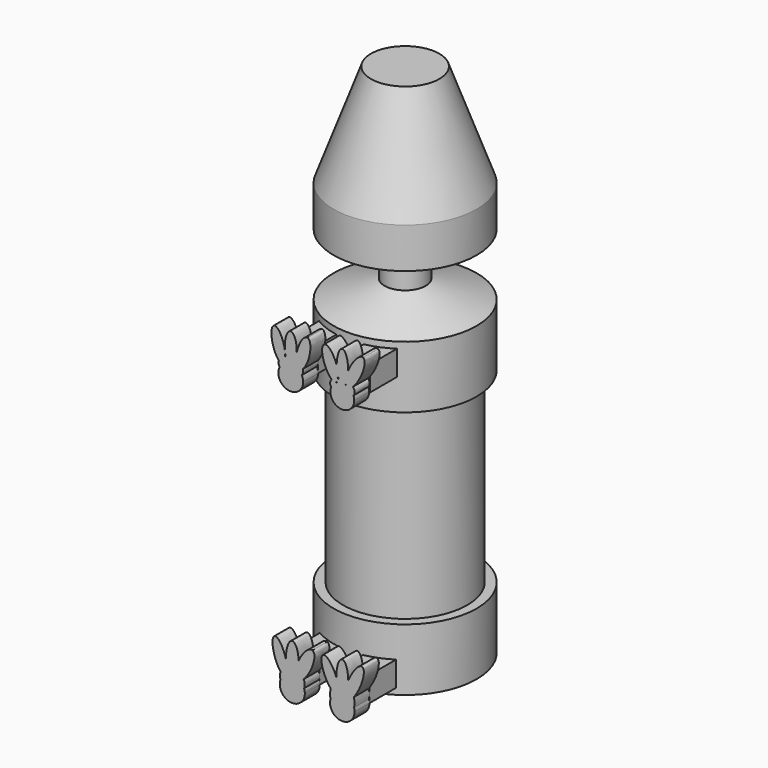
from build123d import *

# Parameters (mm, degrees)
F0_R         = 10
F1_DEPTH     = 40
F2_R         = 11.5
F2_R_2       = 10
F3_DEPTH     = 5
F4_DEPTH     = 5
F5_R         = 11.5
F6_DEPTH     = 5
F7_DEPTH     = 5
F8_W         = 4
F8_H         = 15
F9_DEPTH     = 4
F11_DEPTH    = 3
F12_R        = 11.5
F13_DEPTH    = 3
F13_TAPER    = 70
F14_R        = 3.3
F15_DEPTH    = 5
F16_R        = 11.5
F17_DEPTH    = 25
F18_S5_R     = 3.3
F18_T6_DEPTH = 18
F19_SIZE2    = 16.4848645167
F19_SIZE     = 6
F20_W        = 4
F20_H        = 15
F21_DEPTH    = 4
F23_DEPTH    = 3


# Not quite as in the source:
# - a fillet or chamfer that OpenCascade refuses, or shapes differently, is made with other operations: its cross-section is extruded or revolved along the edge and cut away or added


with BuildPart() as f1:
    # F0 (on Top) → F1 (new body)
    with BuildSketch(Plane.XY):
        Circle(F0_R)
    extrude(amount=F1_DEPTH)

    # F2 (on face) → F3 (join)
    with BuildSketch(Plane.XY.offset(40)):
        Circle(F2_R)
        Circle(F2_R_2, mode=Mode.SUBTRACT)
        Circle(F2_R_2)
    extrude(amount=F3_DEPTH)

    # F4 (add): a face of the model
    f4_faces = [f1.faces().sort_by_distance(p)[0] for p in [
        (-11.1747308807, 0, 40),
    ]]
    extrude(f4_faces, amount=F4_DEPTH)

    # F5 (on face) → F6 (join)
    with BuildSketch(Plane(origin=(0, 0, 0), x_dir=(1, 0, 0), z_dir=(0, 0, -1))):
        Circle(F5_R)
    extrude(amount=F6_DEPTH)

    # F7 (add): a face of the model
    f7_faces = [f1.faces().sort_by_distance(p)[0] for p in [
        (-11.1747308807, 0, 0),
    ]]
    extrude(f7_faces, amount=F7_DEPTH)

    # F8 (on face) → F9 (join)
    with BuildSketch(Plane.XY.offset(40)):
        with Locations((-3.98677176, -7.5)):
            Rectangle(F8_W, F8_H)
        with Locations((4.356082975, -7.5)):
            Rectangle(F8_W, F8_H)
    extrude(amount=F9_DEPTH)

    # F10 (on face) → F11 (join)
    with BuildSketch(Plane.XZ.offset(15)):
        with BuildLine():
            Line((-5.9773173295, 40), (-1.9962261905, 40))
            ThreePointArc((-1.9962261905, 40), (-2.0492726634, 40.4564744405), (-2.2055847885, 40.8886195119))
            add(Edge.make_bspline(
                [(-5.7679587315, 40.8886195119), (-3.98677176, 38.3892921565), (-2.2055847885, 40.8886195119)],
                knots=[0.4528610744, 0.4528610744, 0.4528610744, 2.6887315792, 2.6887315792, 2.6887315792], degree=2, weights=[1, 0.4375399965, 1]))
            ThreePointArc((-5.7679587315, 40.8886195119), (-5.9242708566, 40.4564744405), (-5.9773173295, 40))
        make_face()
        with BuildLine():
            ThreePointArc((-5.9773173295, 40), (-3.98677176, 38.0094544305), (-1.9962261905, 40))
            Line((-1.9962261905, 40), (-5.9773173295, 40))
        make_face()
        with BuildLine():
            add(Edge.make_bspline(
                [(-5.7679587315, 40.8886195119), (-3.98677176, 38.3892921565), (-2.2055847885, 40.8886195119)],
                knots=[0.4528610744, 0.4528610744, 0.4528610744, 2.6887315792, 2.6887315792, 2.6887315792], degree=2, weights=[1, 0.4375399965, 1]))
            ThreePointArc((-2.2055847885, 40.8886195119), (-2.4454357289, 41.2595852109), (-2.7611983029, 41.5685156567))
            add(Edge.make_bspline(
                [(-2.8505101546, 41.6343748739), (-2.8082853314, 41.5943261618), (-2.7611983029, 41.5685156567)],
                knots=[2.9464988752, 2.9464988752, 2.9464988752, 3.055351451, 3.055351451, 3.055351451], degree=2, weights=[1, 0.9985192552, 1]))
            ThreePointArc((-2.8505101546, 41.6343748739), (-3.1356310181, 41.7993974274), (-3.4440645683, 41.9151346084))
            add(Edge.make_bspline(
                [(-4.5294789517, 41.9151346084), (-3.98677176, 40.9549701782), (-3.4440645683, 41.9151346084)],
                knots=[2.5453526146, 2.5453526146, 2.5453526146, 3.7378326925, 3.7378326925, 3.7378326925], degree=2, weights=[1, 0.8274528096, 1]))
            ThreePointArc((-4.5294789517, 41.9151346084), (-5.2570293446, 41.5325525547), (-5.7679587315, 40.8886195119))
        make_face()
        with BuildLine():
            ThreePointArc((-2.7611983029, 41.5685156567), (-2.4454357289, 41.2595852109), (-2.2055847885, 40.8886195119))
            add(Edge.make_bspline(
                [(-2.2055847885, 40.8886195119), (-1.894765034, 41.324755823), (-2.0607312879, 41.7963605451)],
                knots=[2.6887315792, 2.6887315792, 2.6887315792, 3.3774021712, 3.3774021712, 3.3774021712], degree=2, weights=[1, 0.9413000454, 1]))
            add(Edge.make_bspline(
                [(-2.7611983029, 41.5685156567), (-2.4618498874, 41.4044294098), (-2.0607312879, 41.7963605451)],
                knots=[3.055351451, 3.055351451, 3.055351451, 3.7221879744, 3.7221879744, 3.7221879744], degree=2, weights=[1, 0.9449291548, 1]))
        make_face()
        with BuildLine():
            ThreePointArc((-2.8505101546, 41.6343748739), (-2.8053952008, 41.6020677544), (-2.7611983029, 41.5685156567))
            add(Edge.make_bspline(
                [(-2.7611983029, 41.5685156567), (-2.4618498874, 41.4044294098), (-2.0607312879, 41.7963605451)],
                knots=[3.055351451, 3.055351451, 3.055351451, 3.7221879744, 3.7221879744, 3.7221879744], degree=2, weights=[1, 0.9449291548, 1]))
            add(Edge.make_bspline(
                [(-2.0607312879, 41.7963605451), (-2.283512479, 42.4294088862), (-3.1471861713, 42.7053627261)],
                knots=[3.3774021712, 3.3774021712, 3.3774021712, 4.2746981663, 4.2746981663, 4.2746981663], degree=2, weights=[1, 0.9010343537, 1]))
            add(Edge.make_bspline(
                [(-3.1471861713, 42.7053627261), (-3.142060161, 41.910899472), (-2.8505101546, 41.6343748739)],
                knots=[2.2269084938, 2.2269084938, 2.2269084938, 2.9464988752, 2.9464988752, 2.9464988752], degree=2, weights=[1, 0.9359689531, 1]))
        make_face()
        with BuildLine():
            add(Edge.make_bspline(
                [(-5.9676314704, 41.4803815186), (-5.9676314704, 41.1687964649), (-5.7679587315, 40.8886195119)],
                knots=[0, 0, 0, 0.4528610744, 0.4528610744, 0.4528610744], degree=2, weights=[1, 0.9744739478, 1]))
            ThreePointArc((-5.7679587315, 40.8886195119), (-5.2570293446, 41.5325525547), (-4.5294789517, 41.9151346084))
            add(Edge.make_bspline(
                [(-4.816612314, 42.7084544071), (-4.7067779868, 42.2288143047), (-4.5294789517, 41.9151346084)],
                knots=[2.109001467, 2.109001467, 2.109001467, 2.5453526146, 2.5453526146, 2.5453526146], degree=2, weights=[1, 0.9762939688, 1]))
            add(Edge.make_bspline(
                [(-4.816612314, 42.7084544071), (-4.8455679923, 42.6993331341), (-4.8740786521, 42.6895802142)],
                knots=[5.1446550312, 5.1446550312, 5.1446550312, 5.1768492344, 5.1768492344, 5.1768492344], degree=2, weights=[1, 0.9998704445, 1]))
            add(Edge.make_bspline(
                [(-5.9140933068, 41.7926978429), (-4.8978458896, 40.7684913708), (-4.8740786521, 42.6895802142)],
                knots=[2.5752969289, 2.5752969289, 2.5752969289, 4.0574074816, 4.0574074816, 4.0574074816], degree=2, weights=[1, 0.7377565876, 1]))
            add(Edge.make_bspline(
                [(-5.9140933068, 41.7926978429), (-5.9676314704, 41.638678891), (-5.9676314704, 41.4803815186)],
                knots=[6.0501600888, 6.0501600888, 6.0501600888, 6.2831853072, 6.2831853072, 6.2831853072], degree=2, weights=[1, 0.9932200811, 1]))
        make_face()
        with BuildLine():
            add(Edge.make_bspline(
                [(-2.0607312879, 41.7963605451), (-2.283512479, 42.4294088862), (-3.1471861713, 42.7053627261)],
                knots=[3.3774021712, 3.3774021712, 3.3774021712, 4.2746981663, 4.2746981663, 4.2746981663], degree=2, weights=[1, 0.9010343537, 1]))
            add(Edge.make_bspline(
                [(-2.0607312879, 41.7963605451), (-2.0237891501, 41.8324565377), (-1.98677176, 41.8729589071)],
                knots=[3.7221879744, 3.7221879744, 3.7221879744, 3.7859622456, 3.7859622456, 3.7859622456], degree=2, weights=[1, 0.9994916484, 1]))
            Line((-1.98677176, 41.8729589071), (-1.98677176, 44))
            Line((-1.98677176, 44), (-2.9832234994, 44))
            add(Edge.make_bspline(
                [(-2.9832234994, 44), (-3.0041822629, 43.9127168836), (-3.0226179957, 43.8256502166)],
                knots=[1.6769881777, 1.6769881777, 1.6769881777, 1.7474279508, 1.7474279508, 1.7474279508], degree=2, weights=[1, 0.9993798439, 1]))
            add(Edge.make_bspline(
                [(-3.1472064262, 42.7519015627), (-3.0378888264, 43.2516923272), (-3.0226179957, 43.8256502166)],
                knots=[4.1941488137, 4.1941488137, 4.1941488137, 4.6431367414, 4.6431367414, 4.6431367414], degree=2, weights=[1, 0.9749068821, 1]))
            add(Edge.make_bspline(
                [(-3.1472064262, 42.7519015627), (-3.1473353267, 42.7284798246), (-3.1471861713, 42.7053627261)],
                knots=[2.2050180173, 2.2050180173, 2.2050180173, 2.2269084938, 2.2269084938, 2.2269084938], degree=2, weights=[1, 0.9999401015, 1]))
        make_face()
        with BuildLine():
            Line((-1.98677176, 44), (-1.98677176, 41.8729589071))
            add(Edge.make_bspline(
                [(-1.98677176, 41.8729589071), (1.4896787049, 45.6766976511), (-1.289669075, 46.4632548392)],
                knots=[3.7859622456, 3.7859622456, 3.7859622456, 6.2831853072, 6.2831853072, 6.2831853072], degree=2, weights=[1, 0.316639694, 1]))
            add(Edge.make_bspline(
                [(-1.289669075, 46.4632548392), (-2.3216112491, 46.7552951303), (-2.9832234994, 44)],
                knots=[0, 0, 0, 1.6769881777, 1.6769881777, 1.6769881777], degree=2, weights=[1, 0.668583435, 1]))
            Line((-2.9832234994, 44), (-1.98677176, 44))
        make_face()
        with BuildLine():
            ThreePointArc((-3.4440645683, 41.9151346084), (-3.1356310181, 41.7993974274), (-2.8505101546, 41.6343748739))
            add(Edge.make_bspline(
                [(-3.1471861713, 42.7053627261), (-3.142060161, 41.910899472), (-2.8505101546, 41.6343748739)],
                knots=[2.2269084938, 2.2269084938, 2.2269084938, 2.9464988752, 2.9464988752, 2.9464988752], degree=2, weights=[1, 0.9359689531, 1]))
            add(Edge.make_bspline(
                [(-3.1471861713, 42.7053627261), (-3.1520525476, 42.7069175902), (-3.156931206, 42.7084544071)],
                knots=[4.2746981663, 4.2746981663, 4.2746981663, 4.2801229296, 4.2801229296, 4.2801229296], degree=2, weights=[1, 0.9999963215, 1]))
            add(Edge.make_bspline(
                [(-3.4440645683, 41.9151346084), (-3.2667655332, 42.2288143047), (-3.156931206, 42.7084544071)],
                knots=[3.7378326925, 3.7378326925, 3.7378326925, 4.1741838402, 4.1741838402, 4.1741838402], degree=2, weights=[1, 0.9762939688, 1]))
        make_face()
        with BuildLine():
            add(Edge.make_bspline(
                [(-4.816612314, 42.7084544071), (-4.7067779868, 42.2288143047), (-4.5294789517, 41.9151346084)],
                knots=[2.109001467, 2.109001467, 2.109001467, 2.5453526146, 2.5453526146, 2.5453526146], degree=2, weights=[1, 0.9762939688, 1]))
            ThreePointArc((-4.5294789517, 41.9151346084), (-3.98677176, 41.9905455695), (-3.4440645683, 41.9151346084))
            add(Edge.make_bspline(
                [(-3.4440645683, 41.9151346084), (-3.2667655332, 42.2288143047), (-3.156931206, 42.7084544071)],
                knots=[3.7378326925, 3.7378326925, 3.7378326925, 4.1741838402, 4.1741838402, 4.1741838402], degree=2, weights=[1, 0.9762939688, 1]))
            add(Edge.make_bspline(
                [(-3.156931206, 42.7084544071), (-3.98677176, 42.969860898), (-4.816612314, 42.7084544071)],
                knots=[4.2801229296, 4.2801229296, 4.2801229296, 5.1446550312, 5.1446550312, 5.1446550312], degree=2, weights=[1, 0.9080187663, 1]))
        make_face()
        with BuildLine():
            ThreePointArc((-3.4440645683, 41.9151346084), (-3.98677176, 41.9905455695), (-4.5294789517, 41.9151346084))
            add(Edge.make_bspline(
                [(-4.5294789517, 41.9151346084), (-3.98677176, 40.9549701782), (-3.4440645683, 41.9151346084)],
                knots=[2.5453526146, 2.5453526146, 2.5453526146, 3.7378326925, 3.7378326925, 3.7378326925], degree=2, weights=[1, 0.8274528096, 1]))
        make_face()
        with BuildLine():
            Line((-5.98677176, 44), (-5.98677176, 41.8705002355))
            add(Edge.make_bspline(
                [(-5.98677176, 41.8705002355), (-5.9503937124, 41.8292825463), (-5.9140933068, 41.7926978429)],
                knots=[2.509950613, 2.509950613, 2.509950613, 2.5752969289, 2.5752969289, 2.5752969289], degree=2, weights=[1, 0.9994662799, 1]))
            add(Edge.make_bspline(
                [(-4.8740786521, 42.6895802142), (-5.70061296, 42.4068395517), (-5.9140933068, 41.7926978429)],
                knots=[5.1768492344, 5.1768492344, 5.1768492344, 6.0501600888, 6.0501600888, 6.0501600888], degree=2, weights=[1, 0.9061711858, 1]))
            add(Edge.make_bspline(
                [(-4.8740786521, 42.6895802142), (-4.8717422179, 42.8784325276), (-4.8873049815, 43.08528899)],
                knots=[4.0574074816, 4.0574074816, 4.0574074816, 4.2368276577, 4.2368276577, 4.2368276577], degree=2, weights=[1, 0.995978748, 1]))
            add(Edge.make_bspline(
                [(-4.9337451837, 43.4964560034), (-4.9172568336, 43.2857048078), (-4.8873049815, 43.08528899)],
                knots=[1.7720004452, 1.7720004452, 1.7720004452, 1.9423199441, 1.9423199441, 1.9423199441], degree=2, weights=[1, 0.9963760994, 1]))
            add(Edge.make_bspline(
                [(-4.9337451837, 43.4964560034), (-4.9707975236, 43.7455670064), (-5.0291010589, 44)],
                knots=[4.4105111528, 4.4105111528, 4.4105111528, 4.6154032773, 4.6154032773, 4.6154032773], degree=2, weights=[1, 0.9947569901, 1]))
            Line((-5.0291010589, 44), (-5.98677176, 44))
        make_face()
        with BuildLine():
            add(Edge.make_bspline(
                [(-6.643963512, 46.4632548392), (-9.3929519888, 45.7298298908), (-5.98677176, 41.8705002355)],
                knots=[0, 0, 0, 2.509950613, 2.509950613, 2.509950613], degree=2, weights=[1, 0.3105969898, 1]))
            Line((-5.98677176, 41.8705002355), (-5.98677176, 44))
            Line((-5.98677176, 44), (-5.0291010589, 44))
            add(Edge.make_bspline(
                [(-5.0291010589, 44), (-5.6540767082, 46.7273547742), (-6.643963512, 46.4632548392)],
                knots=[4.6154032773, 4.6154032773, 4.6154032773, 6.2831853072, 6.2831853072, 6.2831853072], degree=2, weights=[1, 0.6719993565, 1]))
        make_face()
        with BuildLine():
            add(Edge.make_bspline(
                [(-4.8873049815, 43.08528899), (-4.857995897, 42.889174101), (-4.816612314, 42.7084544071)],
                knots=[1.9423199441, 1.9423199441, 1.9423199441, 2.109001467, 2.109001467, 2.109001467], degree=2, weights=[1, 0.9965291684, 1]))
            add(Edge.make_bspline(
                [(-3.156931206, 42.7084544071), (-3.98677176, 42.969860898), (-4.816612314, 42.7084544071)],
                knots=[4.2801229296, 4.2801229296, 4.2801229296, 5.1446550312, 5.1446550312, 5.1446550312], degree=2, weights=[1, 0.9080187663, 1]))
            add(Edge.make_bspline(
                [(-3.156931206, 42.7084544071), (-3.1519856324, 42.7300514387), (-3.1472064262, 42.7519015627)],
                knots=[4.1741838402, 4.1741838402, 4.1741838402, 4.1941488137, 4.1941488137, 4.1941488137], degree=2, weights=[1, 0.9999501754, 1]))
            add(Edge.make_bspline(
                [(-3.0226179957, 43.8256502166), (-3.1444640287, 43.2502064257), (-3.1472064262, 42.7519015627)],
                knots=[1.7474279508, 1.7474279508, 1.7474279508, 2.2050180173, 2.2050180173, 2.2050180173], degree=2, weights=[1, 0.9739403934, 1]))
            add(Edge.make_bspline(
                [(-3.0226179957, 43.8256502166), (-3.0203013874, 43.9127205048), (-3.0203013874, 44)],
                knots=[4.6431367414, 4.6431367414, 4.6431367414, 4.7123889804, 4.7123889804, 4.7123889804], degree=2, weights=[1, 0.9994005758, 1]))
            Line((-3.0203013874, 44), (-4.9532421326, 44))
            add(Edge.make_bspline(
                [(-4.9532421326, 44), (-4.9532421326, 43.7456625823), (-4.9337451837, 43.4964560034)],
                knots=[1.5707963268, 1.5707963268, 1.5707963268, 1.7720004452, 1.7720004452, 1.7720004452], degree=2, weights=[1, 0.9949438793, 1]))
            add(Edge.make_bspline(
                [(-4.8873049815, 43.08528899), (-4.9023675979, 43.2854976167), (-4.9337451837, 43.4964560034)],
                knots=[4.2368276577, 4.2368276577, 4.2368276577, 4.4105111528, 4.4105111528, 4.4105111528], degree=2, weights=[1, 0.9962316246, 1]))
        make_face()
        with BuildLine():
            add(Edge.make_bspline(
                [(-4.8740786521, 42.6895802142), (-5.70061296, 42.4068395517), (-5.9140933068, 41.7926978429)],
                knots=[5.1768492344, 5.1768492344, 5.1768492344, 6.0501600888, 6.0501600888, 6.0501600888], degree=2, weights=[1, 0.9061711858, 1]))
            add(Edge.make_bspline(
                [(-5.9140933068, 41.7926978429), (-4.8978458896, 40.7684913708), (-4.8740786521, 42.6895802142)],
                knots=[2.5752969289, 2.5752969289, 2.5752969289, 4.0574074816, 4.0574074816, 4.0574074816], degree=2, weights=[1, 0.7377565876, 1]))
        make_face()
        with BuildLine():
            add(Edge.make_bspline(
                [(-3.0226179957, 43.8256502166), (-3.1444640287, 43.2502064257), (-3.1472064262, 42.7519015627)],
                knots=[1.7474279508, 1.7474279508, 1.7474279508, 2.2050180173, 2.2050180173, 2.2050180173], degree=2, weights=[1, 0.9739403934, 1]))
            add(Edge.make_bspline(
                [(-3.1472064262, 42.7519015627), (-3.0378888264, 43.2516923272), (-3.0226179957, 43.8256502166)],
                knots=[4.1941488137, 4.1941488137, 4.1941488137, 4.6431367414, 4.6431367414, 4.6431367414], degree=2, weights=[1, 0.9749068821, 1]))
        make_face()
        with BuildLine():
            add(Edge.make_bspline(
                [(-4.9337451837, 43.4964560034), (-4.9172568336, 43.2857048078), (-4.8873049815, 43.08528899)],
                knots=[1.7720004452, 1.7720004452, 1.7720004452, 1.9423199441, 1.9423199441, 1.9423199441], degree=2, weights=[1, 0.9963760994, 1]))
            add(Edge.make_bspline(
                [(-4.8873049815, 43.08528899), (-4.9023675979, 43.2854976167), (-4.9337451837, 43.4964560034)],
                knots=[4.2368276577, 4.2368276577, 4.2368276577, 4.4105111528, 4.4105111528, 4.4105111528], degree=2, weights=[1, 0.9962316246, 1]))
        make_face()
        with BuildLine():
            Line((-4.9532421326, 44), (-3.0203013874, 44))
            add(Edge.make_bspline(
                [(-3.0203013874, 44), (-3.0203013874, 46.5196184814), (-3.98677176, 46.5196184814)],
                knots=[4.7123889804, 4.7123889804, 4.7123889804, 6.2831853072, 6.2831853072, 6.2831853072], degree=2, weights=[1, 0.7071067812, 1]))
            add(Edge.make_bspline(
                [(-3.98677176, 46.5196184814), (-4.9532421326, 46.5196184814), (-4.9532421326, 44)],
                knots=[0, 0, 0, 1.5707963268, 1.5707963268, 1.5707963268], degree=2, weights=[1, 0.7071067812, 1]))
        make_face()
        with BuildLine():
            ThreePointArc((2.5075891684, 40.7447291667), (3.9450836978, 38.1698190445), (6.213233138, 40.0545075536))
            ThreePointArc((6.213233138, 40.0545075536), (6.1843148739, 40.3862338286), (6.0984325084, 40.7079523497))
            add(Edge.make_bspline(
                [(2.5075891684, 40.7447291667), (4.2399765196, 38.1956403259), (6.0984325084, 40.7079523497)],
                knots=[0.4109771713, 0.4109771713, 0.4109771713, 2.6986743673, 2.6986743673, 2.6986743673], degree=2, weights=[1, 0.4140944549, 1]))
        make_face()
        with BuildLine():
            add(Edge.make_bspline(
                [(2.5075891684, 40.7447291667), (4.2399765196, 38.1956403259), (6.0984325084, 40.7079523497)],
                knots=[0.4109771713, 0.4109771713, 0.4109771713, 2.6986743673, 2.6986743673, 2.6986743673], degree=2, weights=[1, 0.4140944549, 1]))
            ThreePointArc((6.0984325084, 40.7079523497), (5.8668644247, 41.153633472), (5.5274880023, 41.5238753985))
            add(Edge.make_bspline(
                [(4.821201445, 41.6928078856), (4.9899615225, 41.2231285985), (5.5274880023, 41.5238753985)],
                knots=[2.8413853605, 2.8413853605, 2.8413853605, 3.6018285997, 3.6018285997, 3.6018285997], degree=2, weights=[1, 0.9285824095, 1]))
            add(Edge.make_bspline(
                [(3.7232229683, 41.8840052442), (4.2482655074, 40.591386223), (4.821201445, 41.6928078856)],
                knots=[2.4461914573, 2.4461914573, 2.4461914573, 3.7190860479, 3.7190860479, 3.7190860479], degree=2, weights=[1, 0.8042123506, 1]))
            ThreePointArc((3.7232229683, 41.8840052442), (3.600704843, 41.8410315835), (3.4813764244, 41.7898636729))
            add(Edge.make_bspline(
                [(3.1671215791, 41.603902343), (3.3565507705, 41.6181304009), (3.4813764244, 41.7898636729)],
                knots=[3.0271263805, 3.0271263805, 3.0271263805, 3.3897738944, 3.3897738944, 3.3897738944], degree=2, weights=[1, 0.9836058392, 1]))
            ThreePointArc((3.1671215791, 41.603902343), (2.7754169953, 41.2218618947), (2.5075891684, 40.7447291667))
        make_face()
        with BuildLine():
            ThreePointArc((5.5274880023, 41.5238753985), (5.8668644247, 41.153633472), (6.0984325084, 40.7079523497))
            add(Edge.make_bspline(
                [(6.0984325084, 40.7079523497), (6.5518816143, 41.3209373477), (6.0064106373, 41.9022746857)],
                knots=[2.6986743673, 2.6986743673, 2.6986743673, 3.6832450397, 3.6832450397, 3.6832450397], degree=2, weights=[1, 0.881255017, 1]))
            add(Edge.make_bspline(
                [(5.5274880023, 41.5238753985), (5.7513827859, 41.6491448358), (6.0064106373, 41.9022746857)],
                knots=[3.6018285997, 3.6018285997, 3.6018285997, 3.9317502346, 3.9317502346, 3.9317502346], degree=2, weights=[1, 0.9864247904, 1]))
        make_face()
        with BuildLine():
            add(Edge.make_bspline(
                [(2.3433212191, 41.250102222), (2.3433212191, 40.9864381564), (2.5075891684, 40.7447291667)],
                knots=[0, 0, 0, 0.4109771713, 0.4109771713, 0.4109771713], degree=2, weights=[1, 0.9789614077, 1]))
            ThreePointArc((2.5075891684, 40.7447291667), (2.7754169953, 41.2218618947), (3.1671215791, 41.603902343))
            add(Edge.make_bspline(
                [(2.584146034, 41.8557841997), (2.9078881278, 41.5844312755), (3.1671215791, 41.603902343)],
                knots=[2.5354810994, 2.5354810994, 2.5354810994, 3.0271263805, 3.0271263805, 3.0271263805], degree=2, weights=[1, 0.9699374601, 1]))
            add(Edge.make_bspline(
                [(2.584146034, 41.8557841997), (2.3433212191, 41.5726297411), (2.3433212191, 41.250102222)],
                knots=[5.7838967162, 5.7838967162, 5.7838967162, 6.2831853072, 6.2831853072, 6.2831853072], degree=2, weights=[1, 0.9690003631, 1]))
        make_face()
        with BuildLine():
            add(Edge.make_bspline(
                [(4.821201445, 41.6928078856), (4.9899615225, 41.2231285985), (5.5274880023, 41.5238753985)],
                knots=[2.8413853605, 2.8413853605, 2.8413853605, 3.6018285997, 3.6018285997, 3.6018285997], degree=2, weights=[1, 0.9285824095, 1]))
            ThreePointArc((5.5274880023, 41.5238753985), (5.2322423259, 41.7275222236), (4.9042309139, 41.8726103087))
            add(Edge.make_bspline(
                [(4.821201445, 41.6928078856), (4.8644146976, 41.7758817678), (4.9042309139, 41.8726103087)],
                knots=[3.7190860479, 3.7190860479, 3.7190860479, 3.8304532809, 3.8304532809, 3.8304532809], degree=2, weights=[1, 0.998450068, 1]))
        make_face()
        with BuildLine():
            ThreePointArc((4.9042309139, 41.8726103087), (5.2322423259, 41.7275222236), (5.5274880023, 41.5238753985))
            add(Edge.make_bspline(
                [(5.5274880023, 41.5238753985), (5.7513827859, 41.6491448358), (6.0064106373, 41.9022746857)],
                knots=[3.6018285997, 3.6018285997, 3.6018285997, 3.9317502346, 3.9317502346, 3.9317502346], degree=2, weights=[1, 0.9864247904, 1]))
            add(Edge.make_bspline(
                [(6.0064106373, 41.9022746857), (5.6725741879, 42.2580618879), (5.074861157, 42.4177757359)],
                knots=[3.6832450397, 3.6832450397, 3.6832450397, 4.3175648224, 4.3175648224, 4.3175648224], degree=2, weights=[1, 0.9501249917, 1]))
            add(Edge.make_bspline(
                [(4.9042309139, 41.8726103087), (5.0022202749, 42.1106632635), (5.074861157, 42.4177757359)],
                knots=[3.8304532809, 3.8304532809, 3.8304532809, 4.10311441, 4.10311441, 4.10311441], degree=2, weights=[1, 0.990721373, 1]))
        make_face()
        with BuildLine():
            add(Edge.make_bspline(
                [(6.0064106373, 41.9022746857), (5.6725741879, 42.2580618879), (5.074861157, 42.4177757359)],
                knots=[3.6832450397, 3.6832450397, 3.6832450397, 4.3175648224, 4.3175648224, 4.3175648224], degree=2, weights=[1, 0.9501249917, 1]))
            add(Edge.make_bspline(
                [(6.0064106373, 41.9022746857), (9.6800938218, 45.5486171056), (7.6438020915, 46.5904399753)],
                knots=[3.9317502346, 3.9317502346, 3.9317502346, 6.2831853072, 6.2831853072, 6.2831853072], degree=2, weights=[1, 0.384880911, 1]))
            add(Edge.make_bspline(
                [(7.6438020915, 46.5904399753), (6.6110419759, 47.1188284626), (5.2412976718, 43.9492695969)],
                knots=[0, 0, 0, 1.765321057, 1.765321057, 1.765321057], degree=2, weights=[1, 0.6350983189, 1]))
            add(Edge.make_bspline(
                [(5.074861157, 42.4177757359), (5.2380817645, 43.1078428569), (5.2412976718, 43.9492695969)],
                knots=[4.10311441, 4.10311441, 4.10311441, 4.7011133515, 4.7011133515, 4.7011133515], degree=2, weights=[1, 0.9556316875, 1]))
        make_face()
        with BuildLine():
            add(Edge.make_bspline(
                [(2.584146034, 41.8557841997), (2.9078881278, 41.5844312755), (3.1671215791, 41.603902343)],
                knots=[2.5354810994, 2.5354810994, 2.5354810994, 3.0271263805, 3.0271263805, 3.0271263805], degree=2, weights=[1, 0.9699374601, 1]))
            ThreePointArc((3.1671215791, 41.603902343), (3.3198113643, 41.7043821428), (3.4813764244, 41.7898636729))
            add(Edge.make_bspline(
                [(3.4813764244, 41.7898636729), (3.5806086707, 41.9263859166), (3.629197747, 42.1508291202)],
                knots=[3.3897738944, 3.3897738944, 3.3897738944, 3.6792301689, 3.6792301689, 3.6792301689], degree=2, weights=[1, 0.9895451514, 1]))
            add(Edge.make_bspline(
                [(3.5572520688, 42.4177757359), (3.5903934655, 42.2776599222), (3.629197747, 42.1508291202)],
                knots=[2.1800708972, 2.1800708972, 2.1800708972, 2.3050821634, 2.3050821634, 2.3050821634], degree=2, weights=[1, 0.9980471588, 1]))
            add(Edge.make_bspline(
                [(3.5572520688, 42.4177757359), (2.916506235, 42.2465631683), (2.584146034, 41.8557841997)],
                knots=[5.1072131384, 5.1072131384, 5.1072131384, 5.7838967162, 5.7838967162, 5.7838967162], degree=2, weights=[1, 0.9433063611, 1]))
        make_face()
        with BuildLine():
            ThreePointArc((4.7730003113, 41.9113540865), (4.8389613826, 41.8931533692), (4.9042309139, 41.8726103087))
            add(Edge.make_bspline(
                [(4.9042309139, 41.8726103087), (5.0022202749, 42.1106632635), (5.074861157, 42.4177757359)],
                knots=[3.8304532809, 3.8304532809, 3.8304532809, 4.10311441, 4.10311441, 4.10311441], degree=2, weights=[1, 0.990721373, 1]))
            add(Edge.make_bspline(
                [(5.074861157, 42.4177757359), (4.9376625668, 42.45443633), (4.7934464422, 42.4775007606)],
                knots=[4.3175648224, 4.3175648224, 4.3175648224, 4.4679687291, 4.4679687291, 4.4679687291], degree=2, weights=[1, 0.9971736655, 1]))
            add(Edge.make_bspline(
                [(4.7934464422, 42.4775007606), (4.7457322587, 42.1501423241), (4.7730003113, 41.9113540865)],
                knots=[2.371316779, 2.371316779, 2.371316779, 2.6803428621, 2.6803428621, 2.6803428621], degree=2, weights=[1, 0.9880865903, 1]))
        make_face()
        with BuildLine():
            add(Edge.make_bspline(
                [(3.7232229683, 41.8840052442), (4.2482655074, 40.591386223), (4.821201445, 41.6928078856)],
                knots=[2.4461914573, 2.4461914573, 2.4461914573, 3.7190860479, 3.7190860479, 3.7190860479], degree=2, weights=[1, 0.8042123506, 1]))
            add(Edge.make_bspline(
                [(4.7730003113, 41.9113540865), (4.7871277677, 41.7876389657), (4.821201445, 41.6928078856)],
                knots=[2.6803428621, 2.6803428621, 2.6803428621, 2.8413853605, 2.8413853605, 2.8413853605], degree=2, weights=[1, 0.9967599154, 1]))
            ThreePointArc((4.7730003113, 41.9113540865), (4.2462025269, 41.97096041), (3.7232229683, 41.8840052442))
        make_face()
        with BuildLine():
            add(Edge.make_bspline(
                [(5.074861157, 42.4177757359), (4.9376625668, 42.45443633), (4.7934464422, 42.4775007606)],
                knots=[4.3175648224, 4.3175648224, 4.3175648224, 4.4679687291, 4.4679687291, 4.4679687291], degree=2, weights=[1, 0.9971736655, 1]))
            add(Edge.make_bspline(
                [(5.074861157, 42.4177757359), (5.2380817645, 43.1078428569), (5.2412976718, 43.9492695969)],
                knots=[4.10311441, 4.10311441, 4.10311441, 4.7011133515, 4.7011133515, 4.7011133515], degree=2, weights=[1, 0.9556316875, 1]))
            add(Edge.make_bspline(
                [(5.2412976718, 43.9492695969), (4.8892163732, 43.1345610428), (4.7934464422, 42.4775007606)],
                knots=[1.765321057, 1.765321057, 1.765321057, 2.371316779, 2.371316779, 2.371316779], degree=2, weights=[1, 0.9544462691, 1]))
        make_face()
        with BuildLine():
            add(Edge.make_bspline(
                [(3.4813764244, 41.7898636729), (3.5806086707, 41.9263859166), (3.629197747, 42.1508291202)],
                knots=[3.3897738944, 3.3897738944, 3.3897738944, 3.6792301689, 3.6792301689, 3.6792301689], degree=2, weights=[1, 0.9895451514, 1]))
            ThreePointArc((3.4813764244, 41.7898636729), (3.600704843, 41.8410315835), (3.7232229683, 41.8840052442))
            add(Edge.make_bspline(
                [(3.629197747, 42.1508291202), (3.6730146296, 42.0076147594), (3.7232229683, 41.8840052442)],
                knots=[2.3050821634, 2.3050821634, 2.3050821634, 2.4461914573, 2.4461914573, 2.4461914573], degree=2, weights=[1, 0.9975120532, 1]))
        make_face()
        with BuildLine():
            add(Edge.make_bspline(
                [(1.4466231223, 46.4509539306), (-1.5424616006, 45.3146085859), (2.584146034, 41.8557841997)],
                knots=[0, 0, 0, 2.5354810994, 2.5354810994, 2.5354810994], degree=2, weights=[1, 0.2984381177, 1]))
            add(Edge.make_bspline(
                [(3.5572520688, 42.4177757359), (2.916506235, 42.2465631683), (2.584146034, 41.8557841997)],
                knots=[5.1072131384, 5.1072131384, 5.1072131384, 5.7838967162, 5.7838967162, 5.7838967162], degree=2, weights=[1, 0.9433063611, 1]))
            add(Edge.make_bspline(
                [(3.3921621793, 44.1304586166), (3.374574971, 43.1901013686), (3.5572520688, 42.4177757359)],
                knots=[1.5156729511, 1.5156729511, 1.5156729511, 2.1800708972, 2.1800708972, 2.1800708972], degree=2, weights=[1, 0.9453274949, 1]))
            add(Edge.make_bspline(
                [(3.3921621793, 44.1304586166), (2.4892607543, 46.8473282489), (1.4466231223, 46.4509539306)],
                knots=[4.6032690783, 4.6032690783, 4.6032690783, 6.2831853072, 6.2831853072, 6.2831853072], degree=2, weights=[1, 0.6674940151, 1]))
        make_face()
        with BuildLine():
            ThreePointArc((3.7232229683, 41.8840052442), (4.2462025269, 41.97096041), (4.7730003113, 41.9113540865))
            add(Edge.make_bspline(
                [(4.7934464422, 42.4775007606), (4.7457322587, 42.1501423241), (4.7730003113, 41.9113540865)],
                knots=[2.371316779, 2.371316779, 2.371316779, 2.6803428621, 2.6803428621, 2.6803428621], degree=2, weights=[1, 0.9880865903, 1]))
            add(Edge.make_bspline(
                [(4.7934464422, 42.4775007606), (4.2229977271, 42.568732409), (3.6677312476, 42.4448341016)],
                knots=[4.4679687291, 4.4679687291, 4.4679687291, 5.0472552192, 5.0472552192, 5.0472552192], degree=2, weights=[1, 0.9583458294, 1]))
            add(Edge.make_bspline(
                [(3.629197747, 42.1508291202), (3.658173109, 42.2846724359), (3.6677312476, 42.4448341016)],
                knots=[3.6792301689, 3.6792301689, 3.6792301689, 3.8526226984, 3.8526226984, 3.8526226984], degree=2, weights=[1, 0.9962442322, 1]))
            add(Edge.make_bspline(
                [(3.629197747, 42.1508291202), (3.6730146296, 42.0076147594), (3.7232229683, 41.8840052442)],
                knots=[2.3050821634, 2.3050821634, 2.3050821634, 2.4461914573, 2.4461914573, 2.4461914573], degree=2, weights=[1, 0.9975120532, 1]))
        make_face()
        with BuildLine():
            add(Edge.make_bspline(
                [(5.2412976718, 43.9492695969), (4.8892163732, 43.1345610428), (4.7934464422, 42.4775007606)],
                knots=[1.765321057, 1.765321057, 1.765321057, 2.371316779, 2.371316779, 2.371316779], degree=2, weights=[1, 0.9544462691, 1]))
            add(Edge.make_bspline(
                [(5.2412976718, 43.9492695969), (5.251849097, 46.7099994421), (4.3160566129, 46.7099994421)],
                knots=[4.7011133515, 4.7011133515, 4.7011133515, 6.2831853072, 6.2831853072, 6.2831853072], degree=2, weights=[1, 0.7031090278, 1]))
            add(Edge.make_bspline(
                [(4.3160566129, 46.7099994421), (3.4404065268, 46.7099994421), (3.3921621793, 44.1304586166)],
                knots=[0, 0, 0, 1.5156729511, 1.5156729511, 1.5156729511], degree=2, weights=[1, 0.7263248115, 1]))
            add(Edge.make_bspline(
                [(3.6677312476, 42.4448341016), (3.7110602844, 43.1708803574), (3.3921621793, 44.1304586166)],
                knots=[3.8526226984, 3.8526226984, 3.8526226984, 4.6032690783, 4.6032690783, 4.6032690783], degree=2, weights=[1, 0.9303891977, 1]))
            add(Edge.make_bspline(
                [(4.7934464422, 42.4775007606), (4.2229977271, 42.568732409), (3.6677312476, 42.4448341016)],
                knots=[4.4679687291, 4.4679687291, 4.4679687291, 5.0472552192, 5.0472552192, 5.0472552192], degree=2, weights=[1, 0.9583458294, 1]))
        make_face()
        with BuildLine():
            add(Edge.make_bspline(
                [(3.3921621793, 44.1304586166), (3.374574971, 43.1901013686), (3.5572520688, 42.4177757359)],
                knots=[1.5156729511, 1.5156729511, 1.5156729511, 2.1800708972, 2.1800708972, 2.1800708972], degree=2, weights=[1, 0.9453274949, 1]))
            add(Edge.make_bspline(
                [(3.6677312476, 42.4448341016), (3.6118589585, 42.4323671469), (3.5572520688, 42.4177757359)],
                knots=[5.0472552192, 5.0472552192, 5.0472552192, 5.1072131384, 5.1072131384, 5.1072131384], degree=2, weights=[1, 0.9995506646, 1]))
            add(Edge.make_bspline(
                [(3.6677312476, 42.4448341016), (3.7110602844, 43.1708803574), (3.3921621793, 44.1304586166)],
                knots=[3.8526226984, 3.8526226984, 3.8526226984, 4.6032690783, 4.6032690783, 4.6032690783], degree=2, weights=[1, 0.9303891977, 1]))
        make_face()
    extrude(amount=F11_DEPTH)

    # F12 (on face) → F13 (join)
    with BuildSketch(Plane.XY.offset(45)):
        Circle(F12_R)
    extrude(amount=F13_DEPTH, taper=F13_TAPER)

    # F14 (on face) → F15 (join)
    with BuildSketch(Plane.XY.offset(48)):
        Circle(F14_R)
    extrude(amount=F15_DEPTH)

    # F16 (on face) → F17 (join)
    with BuildSketch(Plane.XY.offset(53)):
        Circle(F16_R)
    extrude(amount=F17_DEPTH)

    # F18: chamfer of 2 x 9.409260219 on 1 edges, made by hand


with BuildPart() as f18_tool2:
    # F18_s3 → F18_t4 (revolve)
    with BuildSketch(Plane.XZ):
        Polygon((11.5, 55), (2.090739781, 53), (11.5, 53), align=None)
    revolve(axis=Axis((0, 0, 53), (0, 0, 1)))

    # F18_s5 → F18_t6 (cut, symmetric)
    with BuildSketch(Plane.XY.offset(54)):
        Circle(F18_S5_R)
    extrude(amount=F18_T6_DEPTH, both=True, mode=Mode.SUBTRACT)


with BuildPart() as f1_1:
    add(f1.part)

    # F18_t1: cut F18_tool2
    add(f18_tool2.part, mode=Mode.SUBTRACT)

    # F19
    f19_edges = [f1_1.edges().sort_by_distance(p)[0] for p in [
        (-11.5, 0, 78),
    ]]
    f19_side = f1_1.faces().sort_by_distance((0, 0, 78))[0]
    chamfer(f19_edges, length=F19_SIZE, length2=F19_SIZE2, reference=f19_side)

    # F20 (on face) → F21 (join)
    with BuildSketch(Plane(origin=(0, 0, 0), x_dir=(1, 0, 0), z_dir=(0, 0, -1))):
        with Locations((-3.7374279087, 7.5)):
            Rectangle(F20_W, F20_H)
        with Locations((4.2625720913, 7.5)):
            Rectangle(F20_W, F20_H)
    extrude(amount=F21_DEPTH)

    # F22 (on face) → F23 (join)
    with BuildSketch(Plane.XZ.offset(15)):
        with BuildLine():
            ThreePointArc((-5.7374279087, -3.7773862004), (-3.8489059931, -6.0092609438), (-1.7250768201, -4))
            ThreePointArc((-1.7250768201, -4), (-1.7281669649, -3.8885219157), (-1.7374279087, -3.7773862004))
            Line((-1.7374279087, -3.7773862004), (-1.7374279087, -4))
            Line((-1.7374279087, -4), (-2.3848201371, -4))
            add(Edge.make_bspline(
                [(-5.0900356803, -4), (-3.7374279087, -5.0381021547), (-2.3848201371, -4)],
                knots=[0.8280629734, 0.8280629734, 0.8280629734, 2.3135296802, 2.3135296802, 2.3135296802], degree=2, weights=[1, 0.7366227352, 1]))
            Line((-5.0900356803, -4), (-5.7374279087, -4))
            Line((-5.7374279087, -4), (-5.7374279087, -3.7773862004))
        make_face()
        with BuildLine():
            Line((-1.7374279087, -4), (-1.7374279087, -3.7773862004))
            ThreePointArc((-1.7374279087, -3.7773862004), (-1.7779762673, -3.5416266056), (-1.8462148309, -3.3123445645))
            add(Edge.make_bspline(
                [(-2.3848201371, -4), (-2.0112108326, -3.7132615735), (-1.8462148309, -3.3123445645)],
                knots=[2.3135296802, 2.3135296802, 2.3135296802, 2.8102503859, 2.8102503859, 2.8102503859], degree=2, weights=[1, 0.9693167743, 1]))
            Line((-2.3848201371, -4), (-1.7374279087, -4))
        make_face()
        with BuildLine():
            ThreePointArc((-5.6286409866, -3.3123445645), (-5.6968795501, -3.5416266056), (-5.7374279087, -3.7773862004))
            Line((-5.7374279087, -3.7773862004), (-5.7374279087, -4))
            Line((-5.7374279087, -4), (-5.0900356803, -4))
            add(Edge.make_bspline(
                [(-5.6286409866, -3.3123445645), (-5.4636449848, -3.7132615735), (-5.0900356803, -4)],
                knots=[0.3313422677, 0.3313422677, 0.3313422677, 0.8280629734, 0.8280629734, 0.8280629734], degree=2, weights=[1, 0.9693167743, 1]))
        make_face()
        with BuildLine():
            add(Edge.make_bspline(
                [(-2.3848201371, -4), (-2.0112108326, -3.7132615735), (-1.8462148309, -3.3123445645)],
                knots=[2.3135296802, 2.3135296802, 2.3135296802, 2.8102503859, 2.8102503859, 2.8102503859], degree=2, weights=[1, 0.9693167743, 1]))
            ThreePointArc((-1.8462148309, -3.3123445645), (-2.0921486911, -2.8412881291), (-2.4528086943, -2.4510292521))
            add(Edge.make_bspline(
                [(-3.1754326798, -2.3130553529), (-2.9587377052, -2.7019885879), (-2.4528086943, -2.4510292521)],
                knots=[2.8940215545, 2.8940215545, 2.8940215545, 3.5966021534, 3.5966021534, 3.5966021534], degree=2, weights=[1, 0.9389294901, 1]))
            add(Edge.make_bspline(
                [(-4.4034285095, -2.1010528961), (-3.8189199182, -3.4586151178), (-3.1754326798, -2.3130553529)],
                knots=[2.4324543209, 2.4324543209, 2.4324543209, 3.7233453216, 3.7233453216, 3.7233453216], degree=2, weights=[1, 0.7988318535, 1]))
            ThreePointArc((-4.4034285095, -2.1010528961), (-4.5225074981, -2.1471084916), (-4.638426259, -2.200622642))
            add(Edge.make_bspline(
                [(-5.1300993098, -2.5474080847), (-4.7846720126, -2.6511364219), (-4.638426259, -2.200622642)],
                knots=[2.9165724427, 2.9165724427, 2.9165724427, 3.5750223279, 3.5750223279, 3.5750223279], degree=2, weights=[1, 0.9462932113, 1]))
            ThreePointArc((-5.1300993098, -2.5474080847), (-5.4233271561, -2.9012276708), (-5.6286409866, -3.3123445645))
            add(Edge.make_bspline(
                [(-5.6286409866, -3.3123445645), (-5.4636449848, -3.7132615735), (-5.0900356803, -4)],
                knots=[0.3313422677, 0.3313422677, 0.3313422677, 0.8280629734, 0.8280629734, 0.8280629734], degree=2, weights=[1, 0.9693167743, 1]))
            Line((-5.0900356803, -4), (-2.3848201371, -4))
        make_face()
        with BuildLine():
            ThreePointArc((-2.4528086943, -2.4510292521), (-2.0921486911, -2.8412881291), (-1.8462148309, -3.3123445645))
            add(Edge.make_bspline(
                [(-1.8462148309, -3.3123445645), (-1.7374279087, -3.0480076898), (-1.7374279087, -2.7684655506)],
                knots=[2.8102503859, 2.8102503859, 2.8102503859, 3.1415926536, 3.1415926536, 3.1415926536], degree=2, weights=[1, 0.9863078979, 1]))
            add(Edge.make_bspline(
                [(-1.7374279087, -2.7684655506), (-1.7374279087, -2.3958817544), (-1.9266860478, -2.0585552162)],
                knots=[3.1415926536, 3.1415926536, 3.1415926536, 3.5801365156, 3.5801365156, 3.5801365156], degree=2, weights=[1, 0.9760560769, 1]))
            add(Edge.make_bspline(
                [(-2.4528086943, -2.4510292521), (-2.2043943196, -2.3278066159), (-1.9266860478, -2.0585552162)],
                knots=[3.5966021534, 3.5966021534, 3.5966021534, 3.9526904368, 3.9526904368, 3.9526904368], degree=2, weights=[1, 0.9841919673, 1]))
        make_face()
        with BuildLine():
            add(Edge.make_bspline(
                [(-5.7374279087, -2.7684655506), (-5.7374279087, -3.0480076898), (-5.6286409866, -3.3123445645)],
                knots=[0, 0, 0, 0.3313422677, 0.3313422677, 0.3313422677], degree=2, weights=[1, 0.9863078979, 1]))
            ThreePointArc((-5.6286409866, -3.3123445645), (-5.4233271561, -2.9012276708), (-5.1300993098, -2.5474080847))
            add(Edge.make_bspline(
                [(-5.611214244, -2.1839548447), (-5.3528528052, -2.4805174543), (-5.1300993098, -2.5474080847)],
                knots=[2.4828546925, 2.4828546925, 2.4828546925, 2.9165724427, 2.9165724427, 2.9165724427], degree=2, weights=[1, 0.9765781203, 1]))
            add(Edge.make_bspline(
                [(-5.611214244, -2.1839548447), (-5.7374279087, -2.4666880878), (-5.7374279087, -2.7684655506)],
                knots=[5.9260243369, 5.9260243369, 5.9260243369, 6.2831853072, 6.2831853072, 6.2831853072], degree=2, weights=[1, 0.9840968366, 1]))
        make_face()
        with BuildLine():
            add(Edge.make_bspline(
                [(-3.1754326798, -2.3130553529), (-2.9587377052, -2.7019885879), (-2.4528086943, -2.4510292521)],
                knots=[2.8940215545, 2.8940215545, 2.8940215545, 3.5966021534, 3.5966021534, 3.5966021534], degree=2, weights=[1, 0.9389294901, 1]))
            ThreePointArc((-2.4528086943, -2.4510292521), (-2.7465443241, -2.2485130245), (-3.071427308, -2.1010528961))
            add(Edge.make_bspline(
                [(-3.1754326798, -2.3130553529), (-3.1209323892, -2.2160319214), (-3.071427308, -2.1010528961)],
                knots=[3.7233453216, 3.7233453216, 3.7233453216, 3.8507309862, 3.8507309862, 3.8507309862], degree=2, weights=[1, 0.9979722972, 1]))
        make_face()
        with BuildLine():
            ThreePointArc((-3.071427308, -2.1010528961), (-2.7465443241, -2.2485130245), (-2.4528086943, -2.4510292521))
            add(Edge.make_bspline(
                [(-2.4528086943, -2.4510292521), (-2.2043943196, -2.3278066159), (-1.9266860478, -2.0585552162)],
                knots=[3.5966021534, 3.5966021534, 3.5966021534, 3.9526904368, 3.9526904368, 3.9526904368], degree=2, weights=[1, 0.9841919673, 1]))
            add(Edge.make_bspline(
                [(-1.9266860478, -2.0585552162), (-2.2182695216, -1.5388478776), (-2.8302565336, -1.2784774564)],
                knots=[3.5801365156, 3.5801365156, 3.5801365156, 4.2416043611, 4.2416043611, 4.2416043611], degree=2, weights=[1, 0.9458042662, 1]))
            add(Edge.make_bspline(
                [(-3.071427308, -2.1010528961), (-2.9214915178, -1.7528165014), (-2.8302565336, -1.2784774564)],
                knots=[3.8507309862, 3.8507309862, 3.8507309862, 4.2323654762, 4.2323654762, 4.2323654762], degree=2, weights=[1, 0.9818495632, 1]))
        make_face()
        with BuildLine():
            add(Edge.make_bspline(
                [(-5.0900356803, -4), (-3.7374279087, -5.0381021547), (-2.3848201371, -4)],
                knots=[0.8280629734, 0.8280629734, 0.8280629734, 2.3135296802, 2.3135296802, 2.3135296802], degree=2, weights=[1, 0.7366227352, 1]))
            Line((-2.3848201371, -4), (-5.0900356803, -4))
        make_face()
        with BuildLine():
            add(Edge.make_bspline(
                [(-1.9266860478, -2.0585552162), (-2.2182695216, -1.5388478776), (-2.8302565336, -1.2784774564)],
                knots=[3.5801365156, 3.5801365156, 3.5801365156, 4.2416043611, 4.2416043611, 4.2416043611], degree=2, weights=[1, 0.9458042662, 1]))
            add(Edge.make_bspline(
                [(-1.9266860478, -2.0585552162), (-1.8324101211, -1.967150214), (-1.7374279087, -1.861117524)],
                knots=[3.9526904368, 3.9526904368, 3.9526904368, 4.0747167695, 4.0747167695, 4.0747167695], degree=2, weights=[1, 0.9981392741, 1]))
            Line((-1.7374279087, -1.861117524), (-1.7374279087, 0))
            Line((-1.7374279087, 0), (-2.7146684173, 0))
            add(Edge.make_bspline(
                [(-2.8302565336, -1.2784774564), (-2.7146684173, -0.6775242449), (-2.7146684173, 0)],
                knots=[4.2323654762, 4.2323654762, 4.2323654762, 4.7123889804, 4.7123889804, 4.7123889804], degree=2, weights=[1, 0.9713351813, 1]))
        make_face()
        with BuildLine():
            Line((-1.7374279087, 0), (-1.7374279087, -1.861117524))
            add(Edge.make_bspline(
                [(-1.7374279087, -1.861117524), (1.3496806233, 1.5851532403), (-0.4881575587, 2.5025866926)],
                knots=[4.0747167695, 4.0747167695, 4.0747167695, 6.2831853072, 6.2831853072, 6.2831853072], degree=2, weights=[1, 0.4498184549, 1]))
            add(Edge.make_bspline(
                [(-0.4881575587, 2.5025866926), (-1.459718329, 2.9875817048), (-2.722429161, 0.3404031762)],
                knots=[0, 0, 0, 1.6192128579, 1.6192128579, 1.6192128579], degree=2, weights=[1, 0.689783438, 1]))
            add(Edge.make_bspline(
                [(-2.7146684173, 0), (-2.7146684173, 0.170849796), (-2.722429161, 0.3404031762)],
                knots=[4.7123889804, 4.7123889804, 4.7123889804, 4.8356582752, 4.8356582752, 4.8356582752], degree=2, weights=[1, 0.9981011863, 1]))
            Line((-2.7146684173, 0), (-1.7374279087, 0))
        make_face()
        with BuildLine():
            add(Edge.make_bspline(
                [(-5.611214244, -2.1839548447), (-5.3528528052, -2.4805174543), (-5.1300993098, -2.5474080847)],
                knots=[2.4828546925, 2.4828546925, 2.4828546925, 2.9165724427, 2.9165724427, 2.9165724427], degree=2, weights=[1, 0.9765781203, 1]))
            ThreePointArc((-5.1300993098, -2.5474080847), (-4.8972965512, -2.3555360643), (-4.638426259, -2.200622642))
            add(Edge.make_bspline(
                [(-4.638426259, -2.200622642), (-4.5665524912, -1.9792136642), (-4.558892146, -1.6492601893)],
                knots=[3.5750223279, 3.5750223279, 3.5750223279, 3.9077413515, 3.9077413515, 3.9077413515], degree=2, weights=[1, 0.9861941408, 1]))
            add(Edge.make_bspline(
                [(-4.6445992838, -1.2784774564), (-4.6071728963, -1.4730606752), (-4.558892146, -1.6492601893)],
                knots=[2.050819831, 2.050819831, 2.050819831, 2.2089715437, 2.2089715437, 2.2089715437], degree=2, weights=[1, 0.9968751333, 1]))
            add(Edge.make_bspline(
                [(-4.6445992838, -1.2784774564), (-5.3388608482, -1.5738516595), (-5.611214244, -2.1839548447)],
                knots=[5.1831735996, 5.1831735996, 5.1831735996, 5.9260243369, 5.9260243369, 5.9260243369], degree=2, weights=[1, 0.9318109634, 1]))
        make_face()
        with BuildLine():
            ThreePointArc((-4.638426259, -2.200622642), (-4.8972965512, -2.3555360643), (-5.1300993098, -2.5474080847))
            add(Edge.make_bspline(
                [(-5.1300993098, -2.5474080847), (-4.7846720126, -2.6511364219), (-4.638426259, -2.200622642)],
                knots=[2.9165724427, 2.9165724427, 2.9165724427, 3.5750223279, 3.5750223279, 3.5750223279], degree=2, weights=[1, 0.9462932113, 1]))
        make_face()
        with BuildLine():
            add(Edge.make_bspline(
                [(-5.7374279087, -2.0273700322), (-5.6741393613, -2.1117256564), (-5.611214244, -2.1839548447)],
                knots=[2.3756359074, 2.3756359074, 2.3756359074, 2.4828546925, 2.4828546925, 2.4828546925], degree=2, weights=[1, 0.9985633606, 1]))
            add(Edge.make_bspline(
                [(-4.6445992838, -1.2784774564), (-5.3388608482, -1.5738516595), (-5.611214244, -2.1839548447)],
                knots=[5.1831735996, 5.1831735996, 5.1831735996, 5.9260243369, 5.9260243369, 5.9260243369], degree=2, weights=[1, 0.9318109634, 1]))
            add(Edge.make_bspline(
                [(-4.7581313169, -0.1754564465), (-4.7444306067, -0.7594452584), (-4.6445992838, -1.2784774564)],
                knots=[1.6342156156, 1.6342156156, 1.6342156156, 2.050819831, 2.050819831, 2.050819831], degree=2, weights=[1, 0.9783834473, 1]))
            add(Edge.make_bspline(
                [(-4.7581313169, -0.1754564465), (-4.7806338703, -0.0878310517), (-4.8053767614, 0)],
                knots=[4.5375440599, 4.5375440599, 4.5375440599, 4.6059899368, 4.6059899368, 4.6059899368], degree=2, weights=[1, 0.9994144524, 1]))
            Line((-4.8053767614, 0), (-5.7374279087, 0))
            Line((-5.7374279087, 0), (-5.7374279087, -2.0273700322))
        make_face()
        with BuildLine():
            add(Edge.make_bspline(
                [(-6.5550324507, 2.5509283878), (-8.6649662858, 1.8746681309), (-5.7374279087, -2.0273700322)],
                knots=[0, 0, 0, 2.3756359074, 2.3756359074, 2.3756359074], degree=2, weights=[1, 0.3736847299, 1]))
            Line((-5.7374279087, -2.0273700322), (-5.7374279087, 0))
            Line((-5.7374279087, 0), (-4.8053767614, 0))
            add(Edge.make_bspline(
                [(-4.8053767614, 0), (-5.6093831549, 2.8540208474), (-6.5550324507, 2.5509283878)],
                knots=[4.6059899368, 4.6059899368, 4.6059899368, 6.2831853072, 6.2831853072, 6.2831853072], degree=2, weights=[1, 0.6685063933, 1]))
        make_face()
        with BuildLine():
            add(Edge.make_bspline(
                [(-3.1754326798, -2.3130553529), (-3.1209323892, -2.2160319214), (-3.071427308, -2.1010528961)],
                knots=[3.7233453216, 3.7233453216, 3.7233453216, 3.8507309862, 3.8507309862, 3.8507309862], degree=2, weights=[1, 0.9979722972, 1]))
            ThreePointArc((-3.071427308, -2.1010528961), (-3.1683055877, -2.0698039769), (-3.2666401222, -2.0434939908))
            add(Edge.make_bspline(
                [(-3.2666401222, -2.0434939908), (-3.2372570822, -2.2020903208), (-3.1754326798, -2.3130553529)],
                knots=[2.6856542463, 2.6856542463, 2.6856542463, 2.8940215545, 2.8940215545, 2.8940215545], degree=2, weights=[1, 0.9945777903, 1]))
        make_face()
        with BuildLine():
            ThreePointArc((-3.2666401222, -2.0434939908), (-3.1683055877, -2.0698039769), (-3.071427308, -2.1010528961))
            add(Edge.make_bspline(
                [(-3.071427308, -2.1010528961), (-2.9214915178, -1.7528165014), (-2.8302565336, -1.2784774564)],
                knots=[3.8507309862, 3.8507309862, 3.8507309862, 4.2323654762, 4.2323654762, 4.2323654762], degree=2, weights=[1, 0.9818495632, 1]))
            add(Edge.make_bspline(
                [(-2.8302565336, -1.2784774564), (-3.0224949626, -1.196689445), (-3.231174475, -1.1510470639)],
                knots=[4.2416043611, 4.2416043611, 4.2416043611, 4.456478113, 4.456478113, 4.456478113], degree=2, weights=[1, 0.9942342081, 1]))
            add(Edge.make_bspline(
                [(-3.231174475, -1.1510470639), (-3.3328725111, -1.6860015812), (-3.2666401222, -2.0434939908)],
                knots=[2.2227151144, 2.2227151144, 2.2227151144, 2.6856542463, 2.6856542463, 2.6856542463], degree=2, weights=[1, 0.9733303157, 1]))
        make_face()
        with BuildLine():
            add(Edge.make_bspline(
                [(-4.4034285095, -2.1010528961), (-3.8189199182, -3.4586151178), (-3.1754326798, -2.3130553529)],
                knots=[2.4324543209, 2.4324543209, 2.4324543209, 3.7233453216, 3.7233453216, 3.7233453216], degree=2, weights=[1, 0.7988318535, 1]))
            add(Edge.make_bspline(
                [(-3.2666401222, -2.0434939908), (-3.2372570822, -2.2020903208), (-3.1754326798, -2.3130553529)],
                knots=[2.6856542463, 2.6856542463, 2.6856542463, 2.8940215545, 2.8940215545, 2.8940215545], degree=2, weights=[1, 0.9945777903, 1]))
            ThreePointArc((-3.2666401222, -2.0434939908), (-3.839188744, -1.990223486), (-4.4034285095, -2.1010528961))
        make_face()
        with BuildLine():
            add(Edge.make_bspline(
                [(-2.8302565336, -1.2784774564), (-3.0224949626, -1.196689445), (-3.231174475, -1.1510470639)],
                knots=[4.2416043611, 4.2416043611, 4.2416043611, 4.456478113, 4.456478113, 4.456478113], degree=2, weights=[1, 0.9942342081, 1]))
            add(Edge.make_bspline(
                [(-2.8302565336, -1.2784774564), (-2.7146684173, -0.6775242449), (-2.7146684173, 0)],
                knots=[4.2323654762, 4.2323654762, 4.2323654762, 4.7123889804, 4.7123889804, 4.7123889804], degree=2, weights=[1, 0.9713351813, 1]))
            Line((-2.7146684173, 0), (-2.8744917911, 0))
            add(Edge.make_bspline(
                [(-2.8744917911, 0), (-3.1280175874, -0.6084186596), (-3.231174475, -1.1510470639)],
                knots=[1.7533746794, 1.7533746794, 1.7533746794, 2.2227151144, 2.2227151144, 2.2227151144], degree=2, weights=[1, 0.972591076, 1]))
        make_face()
        with BuildLine():
            add(Edge.make_bspline(
                [(-4.638426259, -2.200622642), (-4.5665524912, -1.9792136642), (-4.558892146, -1.6492601893)],
                knots=[3.5750223279, 3.5750223279, 3.5750223279, 3.9077413515, 3.9077413515, 3.9077413515], degree=2, weights=[1, 0.9861941408, 1]))
            ThreePointArc((-4.638426259, -2.200622642), (-4.5225074981, -2.1471084916), (-4.4034285095, -2.1010528961))
            add(Edge.make_bspline(
                [(-4.558892146, -1.6492601893), (-4.4905245242, -1.8987662897), (-4.4034285095, -2.1010528961)],
                knots=[2.2089715437, 2.2089715437, 2.2089715437, 2.4324543209, 2.4324543209, 2.4324543209], degree=2, weights=[1, 0.9937634243, 1]))
        make_face()
        with BuildLine():
            add(Edge.make_bspline(
                [(-4.5714499182, -1.2489042107), (-4.608384001, -1.263069632), (-4.6445992838, -1.2784774564)],
                knots=[5.1425432296, 5.1425432296, 5.1425432296, 5.1831735996, 5.1831735996, 5.1831735996], degree=2, weights=[1, 0.9997936537, 1]))
            add(Edge.make_bspline(
                [(-4.6445992838, -1.2784774564), (-4.6071728963, -1.4730606752), (-4.558892146, -1.6492601893)],
                knots=[2.050819831, 2.050819831, 2.050819831, 2.2089715437, 2.2089715437, 2.2089715437], degree=2, weights=[1, 0.9968751333, 1]))
            add(Edge.make_bspline(
                [(-4.558892146, -1.6492601893), (-4.5545495509, -1.4622119155), (-4.5714499182, -1.2489042107)],
                knots=[3.9077413515, 3.9077413515, 3.9077413515, 4.0975450158, 4.0975450158, 4.0975450158], degree=2, weights=[1, 0.9955001999, 1]))
        make_face()
        with BuildLine():
            add(Edge.make_bspline(
                [(-4.7581313169, -0.1754564465), (-4.7444306067, -0.7594452584), (-4.6445992838, -1.2784774564)],
                knots=[1.6342156156, 1.6342156156, 1.6342156156, 2.050819831, 2.050819831, 2.050819831], degree=2, weights=[1, 0.9783834473, 1]))
            add(Edge.make_bspline(
                [(-4.5714499182, -1.2489042107), (-4.608384001, -1.263069632), (-4.6445992838, -1.2784774564)],
                knots=[5.1425432296, 5.1425432296, 5.1425432296, 5.1831735996, 5.1831735996, 5.1831735996], degree=2, weights=[1, 0.9997936537, 1]))
            add(Edge.make_bspline(
                [(-4.5714499182, -1.2489042107), (-4.611152938, -0.7477932059), (-4.7581313169, -0.1754564465)],
                knots=[4.0975450158, 4.0975450158, 4.0975450158, 4.5375440599, 4.5375440599, 4.5375440599], degree=2, weights=[1, 0.9758975536, 1]))
        make_face()
        with BuildLine():
            ThreePointArc((-4.4034285095, -2.1010528961), (-3.839188744, -1.990223486), (-3.2666401222, -2.0434939908))
            add(Edge.make_bspline(
                [(-3.231174475, -1.1510470639), (-3.3328725111, -1.6860015812), (-3.2666401222, -2.0434939908)],
                knots=[2.2227151144, 2.2227151144, 2.2227151144, 2.6856542463, 2.6856542463, 2.6856542463], degree=2, weights=[1, 0.9733303157, 1]))
            add(Edge.make_bspline(
                [(-3.231174475, -1.1510470639), (-3.9222169423, -0.9999022616), (-4.5714499182, -1.2489042107)],
                knots=[4.456478113, 4.456478113, 4.456478113, 5.1425432296, 5.1425432296, 5.1425432296], degree=2, weights=[1, 0.941739013, 1]))
            add(Edge.make_bspline(
                [(-4.558892146, -1.6492601893), (-4.5545495509, -1.4622119155), (-4.5714499182, -1.2489042107)],
                knots=[3.9077413515, 3.9077413515, 3.9077413515, 4.0975450158, 4.0975450158, 4.0975450158], degree=2, weights=[1, 0.9955001999, 1]))
            add(Edge.make_bspline(
                [(-4.558892146, -1.6492601893), (-4.4905245242, -1.8987662897), (-4.4034285095, -2.1010528961)],
                knots=[2.2089715437, 2.2089715437, 2.2089715437, 2.4324543209, 2.4324543209, 2.4324543209], degree=2, weights=[1, 0.9937634243, 1]))
        make_face()
        with BuildLine():
            Line((-2.8744917911, 0), (-2.7146684173, 0))
            add(Edge.make_bspline(
                [(-2.7146684173, 0), (-2.7146684173, 0.170849796), (-2.722429161, 0.3404031762)],
                knots=[4.7123889804, 4.7123889804, 4.7123889804, 4.8356582752, 4.8356582752, 4.8356582752], degree=2, weights=[1, 0.9981011863, 1]))
            add(Edge.make_bspline(
                [(-2.722429161, 0.3404031762), (-2.8032493215, 0.1709697729), (-2.8744917911, 0)],
                knots=[1.6192128579, 1.6192128579, 1.6192128579, 1.7533746794, 1.7533746794, 1.7533746794], degree=2, weights=[1, 0.9977509193, 1]))
        make_face()
        with BuildLine():
            add(Edge.make_bspline(
                [(-3.231174475, -1.1510470639), (-3.9222169423, -0.9999022616), (-4.5714499182, -1.2489042107)],
                knots=[4.456478113, 4.456478113, 4.456478113, 5.1425432296, 5.1425432296, 5.1425432296], degree=2, weights=[1, 0.941739013, 1]))
            add(Edge.make_bspline(
                [(-2.8744917911, 0), (-3.1280175874, -0.6084186596), (-3.231174475, -1.1510470639)],
                knots=[1.7533746794, 1.7533746794, 1.7533746794, 2.2227151144, 2.2227151144, 2.2227151144], degree=2, weights=[1, 0.972591076, 1]))
            Line((-2.8744917911, 0), (-4.7601874001, 0))
            add(Edge.make_bspline(
                [(-4.7601874001, 0), (-4.7601874001, -0.0878164933), (-4.7581313169, -0.1754564465)],
                knots=[1.5707963268, 1.5707963268, 1.5707963268, 1.6342156156, 1.6342156156, 1.6342156156], degree=2, weights=[1, 0.9994972914, 1]))
            add(Edge.make_bspline(
                [(-4.5714499182, -1.2489042107), (-4.611152938, -0.7477932059), (-4.7581313169, -0.1754564465)],
                knots=[4.0975450158, 4.0975450158, 4.0975450158, 4.5375440599, 4.5375440599, 4.5375440599], degree=2, weights=[1, 0.9758975536, 1]))
        make_face()
        with BuildLine():
            add(Edge.make_bspline(
                [(-2.722429161, 0.3404031762), (-2.8032493215, 0.1709697729), (-2.8744917911, 0)],
                knots=[1.6192128579, 1.6192128579, 1.6192128579, 1.7533746794, 1.7533746794, 1.7533746794], degree=2, weights=[1, 0.9977509193, 1]))
            add(Edge.make_bspline(
                [(-2.722429161, 0.3404031762), (-2.8335656636, 2.7684655506), (-3.7374279087, 2.7684655506)],
                knots=[4.8356582752, 4.8356582752, 4.8356582752, 6.2831853072, 6.2831853072, 6.2831853072], degree=2, weights=[1, 0.7493188059, 1]))
            add(Edge.make_bspline(
                [(-3.7374279087, 2.7684655506), (-4.7601874001, 2.7684655506), (-4.7601874001, 0)],
                knots=[0, 0, 0, 1.5707963268, 1.5707963268, 1.5707963268], degree=2, weights=[1, 0.7071067812, 1]))
            Line((-4.7601874001, 0), (-2.8744917911, 0))
        make_face()
        with BuildLine():
            ThreePointArc((2.4064365087, -3.4498529202), (4.0198118013, -5.9499233682), (6.2672839231, -4))
            ThreePointArc((6.2672839231, -4), (6.2475872915, -3.722147878), (6.188891338, -3.4498529202))
            add(Edge.make_bspline(
                [(2.4064365087, -3.4498529202), (2.7950472686, -5.4031430109), (4.2976639234, -5.4031430109), (5.8002805781, -5.4031430109), (6.188891338, -3.4498529202)],
                knots=[4.973985091, 4.973985091, 4.973985091, 6.2831853072, 6.2831853072, 7.5923855234, 7.5923855234, 7.5923855234], degree=2, weights=[1, 0.7932914625, 1, 0.7932914625, 1]))
        make_face()
        with BuildLine():
            add(Edge.make_bspline(
                [(2.4064365087, -3.4498529202), (2.7950472686, -5.4031430109), (4.2976639234, -5.4031430109), (5.8002805781, -5.4031430109), (6.188891338, -3.4498529202)],
                knots=[4.973985091, 4.973985091, 4.973985091, 6.2831853072, 6.2831853072, 7.5923855234, 7.5923855234, 7.5923855234], degree=2, weights=[1, 0.7932914625, 1, 0.7932914625, 1]))
            ThreePointArc((6.188891338, -3.4498529202), (5.9662683004, -2.9534999396), (5.6163613501, -2.5369757213))
            add(Edge.make_bspline(
                [(4.7365225915, -2.4627083541), (4.9127784824, -3.124664224), (5.6163613501, -2.5369757213)],
                knots=[2.7889443234, 2.7889443234, 2.7889443234, 3.7161510021, 3.7161510021, 3.7161510021], degree=2, weights=[1, 0.8944469881, 1]))
            add(Edge.make_bspline(
                [(3.6834127858, -2.1286105474), (4.1716517184, -3.2986719446), (4.7365225915, -2.4627083541)],
                knots=[2.4478798748, 2.4478798748, 2.4478798748, 3.6160141155, 3.6160141155, 3.6160141155], degree=2, weights=[1, 0.8342268586, 1]))
            ThreePointArc((3.6834127858, -2.1286105474), (3.6568935537, -2.137524154), (3.6305036058, -2.1468135404))
            add(Edge.make_bspline(
                [(3.10345566, -2.4337083391), (3.4883515779, -2.554664474), (3.6305036058, -2.1468135404)],
                knots=[2.8412285078, 2.8412285078, 2.8412285078, 3.4963017358, 3.4963017358, 3.4963017358], degree=2, weights=[1, 0.9468377154, 1]))
            ThreePointArc((3.10345566, -2.4337083391), (2.6734361735, -2.8858693254), (2.4064365087, -3.4498529202))
        make_face()
        with BuildLine():
            ThreePointArc((5.6163613501, -2.5369757213), (5.9662683004, -2.9534999396), (6.188891338, -3.4498529202))
            add(Edge.make_bspline(
                [(6.188891338, -3.4498529202), (6.3392092085, -2.6943040854), (6.1588206674, -1.950768539)],
                knots=[1.3092002162, 1.3092002162, 1.3092002162, 1.8863674435, 1.8863674435, 1.8863674435], degree=2, weights=[1, 0.958647933, 1]))
            add(Edge.make_bspline(
                [(5.6163613501, -2.5369757213), (5.8759001604, -2.3201882158), (6.1588206674, -1.950768539)],
                knots=[3.7161510021, 3.7161510021, 3.7161510021, 4.0808936052, 4.0808936052, 4.0808936052], degree=2, weights=[1, 0.983416394, 1]))
        make_face()
        with BuildLine():
            add(Edge.make_bspline(
                [(2.3398278281, -2.7684655506), (2.3398278281, -3.115054996), (2.4064365087, -3.4498529202)],
                knots=[4.7123889804, 4.7123889804, 4.7123889804, 4.973985091, 4.973985091, 4.973985091], degree=2, weights=[1, 0.9914581228, 1]))
            ThreePointArc((2.4064365087, -3.4498529202), (2.6734361735, -2.8858693254), (3.10345566, -2.4337083391))
            add(Edge.make_bspline(
                [(2.4395087422, -1.9384985647), (2.8034524388, -2.339430306), (3.10345566, -2.4337083391)],
                knots=[2.3234472548, 2.3234472548, 2.3234472548, 2.8412285078, 2.8412285078, 2.8412285078], degree=2, weights=[1, 0.9666745818, 1]))
            add(Edge.make_bspline(
                [(2.4395087422, -1.9384985647), (2.3398278281, -2.3426419035), (2.3398278281, -2.7684655506)],
                knots=[4.3919148958, 4.3919148958, 4.3919148958, 4.7123889804, 4.7123889804, 4.7123889804], degree=2, weights=[1, 0.9871894905, 1]))
        make_face()
        with BuildLine():
            add(Edge.make_bspline(
                [(4.7365225915, -2.4627083541), (4.9127784824, -3.124664224), (5.6163613501, -2.5369757213)],
                knots=[2.7889443234, 2.7889443234, 2.7889443234, 3.7161510021, 3.7161510021, 3.7161510021], degree=2, weights=[1, 0.8944469881, 1]))
            ThreePointArc((5.6163613501, -2.5369757213), (5.2854711246, -2.295992994), (4.9119150609, -2.1286105474))
            add(Edge.make_bspline(
                [(4.7365225915, -2.4627083541), (4.830600243, -2.3234809747), (4.9119150609, -2.1286105474)],
                knots=[3.6160141155, 3.6160141155, 3.6160141155, 3.8353054324, 3.8353054324, 3.8353054324], degree=2, weights=[1, 0.9939949346, 1]))
        make_face()
        with BuildLine():
            ThreePointArc((4.9119150609, -2.1286105474), (5.2854711246, -2.295992994), (5.6163613501, -2.5369757213))
            add(Edge.make_bspline(
                [(5.6163613501, -2.5369757213), (5.8759001604, -2.3201882158), (6.1588206674, -1.950768539)],
                knots=[3.7161510021, 3.7161510021, 3.7161510021, 4.0808936052, 4.0808936052, 4.0808936052], degree=2, weights=[1, 0.983416394, 1]))
            add(Edge.make_bspline(
                [(6.1588206674, -1.950768539), (5.9195509331, -0.9645332068), (5.244829564, -0.4626258724)],
                knots=[1.8863674435, 1.8863674435, 1.8863674435, 2.6366218513, 2.6366218513, 2.6366218513], degree=2, weights=[1, 0.9304610231, 1]))
            add(Edge.make_bspline(
                [(4.9119150609, -2.1286105474), (5.1853927403, -1.4732230839), (5.244829564, -0.4626258724)],
                knots=[3.8353054324, 3.8353054324, 3.8353054324, 4.544495807, 4.544495807, 4.544495807], degree=2, weights=[1, 0.937787121, 1]))
        make_face()
        with BuildLine():
            add(Edge.make_bspline(
                [(6.1588206674, -1.950768539), (5.9195509331, -0.9645332068), (5.244829564, -0.4626258724)],
                knots=[1.8863674435, 1.8863674435, 1.8863674435, 2.6366218513, 2.6366218513, 2.6366218513], degree=2, weights=[1, 0.9304610231, 1]))
            add(Edge.make_bspline(
                [(6.1588206674, -1.950768539), (9.1815336782, 1.9960986414), (7.5123822317, 2.7684655506)],
                knots=[4.0808936052, 4.0808936052, 4.0808936052, 6.2831853072, 6.2831853072, 6.2831853072], degree=2, weights=[1, 0.452574633, 1]))
            add(Edge.make_bspline(
                [(7.5123822317, 2.7684655506), (6.5736873096, 3.2028281108), (5.2576222566, 0.1068160448)],
                knots=[0, 0, 0, 1.6732433396, 1.6732433396, 1.6732433396], degree=2, weights=[1, 0.6699746625, 1]))
            add(Edge.make_bspline(
                [(5.244829564, -0.4626258724), (5.2614626925, -0.1798147779), (5.2576222566, 0.1068160448)],
                knots=[4.544495807, 4.544495807, 4.544495807, 4.7509816819, 4.7509816819, 4.7509816819], degree=2, weights=[1, 0.9946751803, 1]))
        make_face()
        with BuildLine():
            add(Edge.make_bspline(
                [(2.4395087422, -1.9384985647), (2.8034524388, -2.339430306), (3.10345566, -2.4337083391)],
                knots=[2.3234472548, 2.3234472548, 2.3234472548, 2.8412285078, 2.8412285078, 2.8412285078], degree=2, weights=[1, 0.9666745818, 1]))
            ThreePointArc((3.10345566, -2.4337083391), (3.3559896671, -2.2700715222), (3.6305036058, -2.1468135404))
            add(Edge.make_bspline(
                [(3.6305036058, -2.1468135404), (3.6447541393, -2.1059270789), (3.6559241704, -2.0601596247)],
                knots=[3.4963017358, 3.4963017358, 3.4963017358, 3.5643992614, 3.5643992614, 3.5643992614], degree=2, weights=[1, 0.9994203969, 1]))
            add(Edge.make_bspline(
                [(3.3504982827, -0.4626258724), (3.4065069754, -1.4149349816), (3.6559241704, -2.0601596247)],
                knots=[1.7386895002, 1.7386895002, 1.7386895002, 2.4100610696, 2.4100610696, 2.4100610696], degree=2, weights=[1, 0.9441846227, 1]))
            add(Edge.make_bspline(
                [(3.3504982827, -0.4626258724), (2.680624131, -0.9609274903), (2.4395087422, -1.9384985647)],
                knots=[3.6465634559, 3.6465634559, 3.6465634559, 4.3919148958, 4.3919148958, 4.3919148958], degree=2, weights=[1, 0.9313564277, 1]))
        make_face()
        with BuildLine():
            ThreePointArc((3.6305036058, -2.1468135404), (3.3559896671, -2.2700715222), (3.10345566, -2.4337083391))
            add(Edge.make_bspline(
                [(3.10345566, -2.4337083391), (3.4883515779, -2.554664474), (3.6305036058, -2.1468135404)],
                knots=[2.8412285078, 2.8412285078, 2.8412285078, 3.4963017358, 3.4963017358, 3.4963017358], degree=2, weights=[1, 0.9468377154, 1]))
        make_face()
        with BuildLine():
            add(Edge.make_bspline(
                [(4.7365225915, -2.4627083541), (4.830600243, -2.3234809747), (4.9119150609, -2.1286105474)],
                knots=[3.6160141155, 3.6160141155, 3.6160141155, 3.8353054324, 3.8353054324, 3.8353054324], degree=2, weights=[1, 0.9939949346, 1]))
            ThreePointArc((4.9119150609, -2.1286105474), (4.8045852249, -2.0967307764), (4.695617309, -2.071001284))
            add(Edge.make_bspline(
                [(4.695617309, -2.071001284), (4.6934027755, -2.3007653115), (4.7365225915, -2.4627083541)],
                knots=[2.5455370649, 2.5455370649, 2.5455370649, 2.7889443234, 2.7889443234, 2.7889443234], degree=2, weights=[1, 0.99260325, 1]))
        make_face()
        with BuildLine():
            ThreePointArc((4.695617309, -2.071001284), (4.8045852249, -2.0967307764), (4.9119150609, -2.1286105474))
            add(Edge.make_bspline(
                [(4.9119150609, -2.1286105474), (5.1853927403, -1.4732230839), (5.244829564, -0.4626258724)],
                knots=[3.8353054324, 3.8353054324, 3.8353054324, 4.544495807, 4.544495807, 4.544495807], degree=2, weights=[1, 0.937787121, 1]))
            add(Edge.make_bspline(
                [(5.244829564, -0.4626258724), (5.1626956017, -0.4015285959), (5.0765956197, -0.3512833133)],
                knots=[2.6366218513, 2.6366218513, 2.6366218513, 2.7324167747, 2.7324167747, 2.7324167747], degree=2, weights=[1, 0.9988531359, 1]))
            add(Edge.make_bspline(
                [(5.0765956197, -0.3512833133), (4.7023099655, -1.3766194903), (4.695617309, -2.071001284)],
                knots=[1.8374217991, 1.8374217991, 1.8374217991, 2.5455370649, 2.5455370649, 2.5455370649], degree=2, weights=[1, 0.9379736302, 1]))
        make_face()
        with BuildLine():
            add(Edge.make_bspline(
                [(3.6834127858, -2.1286105474), (4.1716517184, -3.2986719446), (4.7365225915, -2.4627083541)],
                knots=[2.4478798748, 2.4478798748, 2.4478798748, 3.6160141155, 3.6160141155, 3.6160141155], degree=2, weights=[1, 0.8342268586, 1]))
            add(Edge.make_bspline(
                [(4.695617309, -2.071001284), (4.6934027755, -2.3007653115), (4.7365225915, -2.4627083541)],
                knots=[2.5455370649, 2.5455370649, 2.5455370649, 2.7889443234, 2.7889443234, 2.7889443234], degree=2, weights=[1, 0.99260325, 1]))
            ThreePointArc((4.695617309, -2.071001284), (4.1857448179, -2.0335623434), (3.6834127858, -2.1286105474))
        make_face()
        with BuildLine():
            add(Edge.make_bspline(
                [(5.244829564, -0.4626258724), (5.1626956017, -0.4015285959), (5.0765956197, -0.3512833133)],
                knots=[2.6366218513, 2.6366218513, 2.6366218513, 2.7324167747, 2.7324167747, 2.7324167747], degree=2, weights=[1, 0.9988531359, 1]))
            add(Edge.make_bspline(
                [(5.244829564, -0.4626258724), (5.2614626925, -0.1798147779), (5.2576222566, 0.1068160448)],
                knots=[4.544495807, 4.544495807, 4.544495807, 4.7509816819, 4.7509816819, 4.7509816819], degree=2, weights=[1, 0.9946751803, 1]))
            add(Edge.make_bspline(
                [(5.2576222566, 0.1068160448), (5.1599051974, -0.1230610374), (5.0765956197, -0.3512833133)],
                knots=[1.6732433396, 1.6732433396, 1.6732433396, 1.8374217991, 1.8374217991, 1.8374217991], degree=2, weights=[1, 0.9966325708, 1]))
        make_face()
        with BuildLine():
            add(Edge.make_bspline(
                [(1.2279704679, 2.4300741497), (-0.7303660878, 1.5535345351), (2.4395087422, -1.9384985647)],
                knots=[0, 0, 0, 2.3234472548, 2.3234472548, 2.3234472548], degree=2, weights=[1, 0.39775871, 1]))
            add(Edge.make_bspline(
                [(3.3504982827, -0.4626258724), (2.680624131, -0.9609274903), (2.4395087422, -1.9384985647)],
                knots=[3.6465634559, 3.6465634559, 3.6465634559, 4.3919148958, 4.3919148958, 4.3919148958], degree=2, weights=[1, 0.9313564277, 1]))
            add(Edge.make_bspline(
                [(3.337082307, -0.0383216633), (3.3381086071, -0.251965699), (3.3504982827, -0.4626258724)],
                knots=[1.5846389723, 1.5846389723, 1.5846389723, 1.7386895002, 1.7386895002, 1.7386895002], degree=2, weights=[1, 0.9970350207, 1]))
            add(Edge.make_bspline(
                [(3.337082307, -0.0383216633), (2.2358364334, 2.8811888688), (1.2279704679, 2.4300741497)],
                knots=[4.5416881204, 4.5416881204, 4.5416881204, 6.2831853072, 6.2831853072, 6.2831853072], degree=2, weights=[1, 0.644254195, 1]))
        make_face()
        with BuildLine():
            ThreePointArc((3.6834127858, -2.1286105474), (4.1857448179, -2.0335623434), (4.695617309, -2.071001284))
            add(Edge.make_bspline(
                [(5.0765956197, -0.3512833133), (4.7023099655, -1.3766194903), (4.695617309, -2.071001284)],
                knots=[1.8374217991, 1.8374217991, 1.8374217991, 2.5455370649, 2.5455370649, 2.5455370649], degree=2, weights=[1, 0.9379736302, 1]))
            add(Edge.make_bspline(
                [(5.0765956197, -0.3512833133), (4.2614715661, 0.1243978364), (3.4587085157, -0.3879388353)],
                knots=[2.7324167747, 2.7324167747, 2.7324167747, 3.584437441, 3.584437441, 3.584437441], degree=2, weights=[1, 0.9106216867, 1]))
            add(Edge.make_bspline(
                [(3.6559241704, -2.0601596247), (3.8012866979, -1.4645594166), (3.4587085157, -0.3879388353)],
                knots=[3.5643992614, 3.5643992614, 3.5643992614, 4.3988838404, 4.3988838404, 4.3988838404], degree=2, weights=[1, 0.9142099522, 1]))
            add(Edge.make_bspline(
                [(3.6559241704, -2.0601596247), (3.6694438751, -2.0951341444), (3.6834127858, -2.1286105474)],
                knots=[2.4100610696, 2.4100610696, 2.4100610696, 2.4478798748, 2.4478798748, 2.4478798748], degree=2, weights=[1, 0.9998212226, 1]))
        make_face()
        with BuildLine():
            add(Edge.make_bspline(
                [(5.2576222566, 0.1068160448), (5.1599051974, -0.1230610374), (5.0765956197, -0.3512833133)],
                knots=[1.6732433396, 1.6732433396, 1.6732433396, 1.8374217991, 1.8374217991, 1.8374217991], degree=2, weights=[1, 0.9966325708, 1]))
            add(Edge.make_bspline(
                [(5.2576222566, 0.1068160448), (5.221960027, 2.7684655506), (4.2976639234, 2.7684655506)],
                knots=[4.7509816819, 4.7509816819, 4.7509816819, 6.2831853072, 6.2831853072, 6.2831853072], degree=2, weights=[1, 0.7206188737, 1]))
            add(Edge.make_bspline(
                [(4.2976639234, 2.7684655506), (3.3235991036, 2.7684655506), (3.337082307, -0.0383216633)],
                knots=[0, 0, 0, 1.5846389723, 1.5846389723, 1.5846389723], degree=2, weights=[1, 0.7021957692, 1]))
            add(Edge.make_bspline(
                [(3.4587085157, -0.3879388353), (3.4034317579, -0.2142205478), (3.337082307, -0.0383216633)],
                knots=[4.3988838404, 4.3988838404, 4.3988838404, 4.5416881204, 4.5416881204, 4.5416881204], degree=2, weights=[1, 0.99745195, 1]))
            add(Edge.make_bspline(
                [(5.0765956197, -0.3512833133), (4.2614715661, 0.1243978364), (3.4587085157, -0.3879388353)],
                knots=[2.7324167747, 2.7324167747, 2.7324167747, 3.584437441, 3.584437441, 3.584437441], degree=2, weights=[1, 0.9106216867, 1]))
        make_face()
        with BuildLine():
            add(Edge.make_bspline(
                [(3.3504982827, -0.4626258724), (3.4065069754, -1.4149349816), (3.6559241704, -2.0601596247)],
                knots=[1.7386895002, 1.7386895002, 1.7386895002, 2.4100610696, 2.4100610696, 2.4100610696], degree=2, weights=[1, 0.9441846227, 1]))
            add(Edge.make_bspline(
                [(3.6559241704, -2.0601596247), (3.8012866979, -1.4645594166), (3.4587085157, -0.3879388353)],
                knots=[3.5643992614, 3.5643992614, 3.5643992614, 4.3988838404, 4.3988838404, 4.3988838404], degree=2, weights=[1, 0.9142099522, 1]))
            add(Edge.make_bspline(
                [(3.4587085157, -0.3879388353), (3.4037411211, -0.4230199367), (3.3504982827, -0.4626258724)],
                knots=[3.584437441, 3.584437441, 3.584437441, 3.6465634559, 3.6465634559, 3.6465634559], degree=2, weights=[1, 0.9995175836, 1]))
        make_face()
        with BuildLine():
            add(Edge.make_bspline(
                [(3.337082307, -0.0383216633), (3.3381086071, -0.251965699), (3.3504982827, -0.4626258724)],
                knots=[1.5846389723, 1.5846389723, 1.5846389723, 1.7386895002, 1.7386895002, 1.7386895002], degree=2, weights=[1, 0.9970350207, 1]))
            add(Edge.make_bspline(
                [(3.4587085157, -0.3879388353), (3.4037411211, -0.4230199367), (3.3504982827, -0.4626258724)],
                knots=[3.584437441, 3.584437441, 3.584437441, 3.6465634559, 3.6465634559, 3.6465634559], degree=2, weights=[1, 0.9995175836, 1]))
            add(Edge.make_bspline(
                [(3.4587085157, -0.3879388353), (3.4034317579, -0.2142205478), (3.337082307, -0.0383216633)],
                knots=[4.3988838404, 4.3988838404, 4.3988838404, 4.5416881204, 4.5416881204, 4.5416881204], degree=2, weights=[1, 0.99745195, 1]))
        make_face()
    extrude(amount=F23_DEPTH)


solid = f1_1.part
